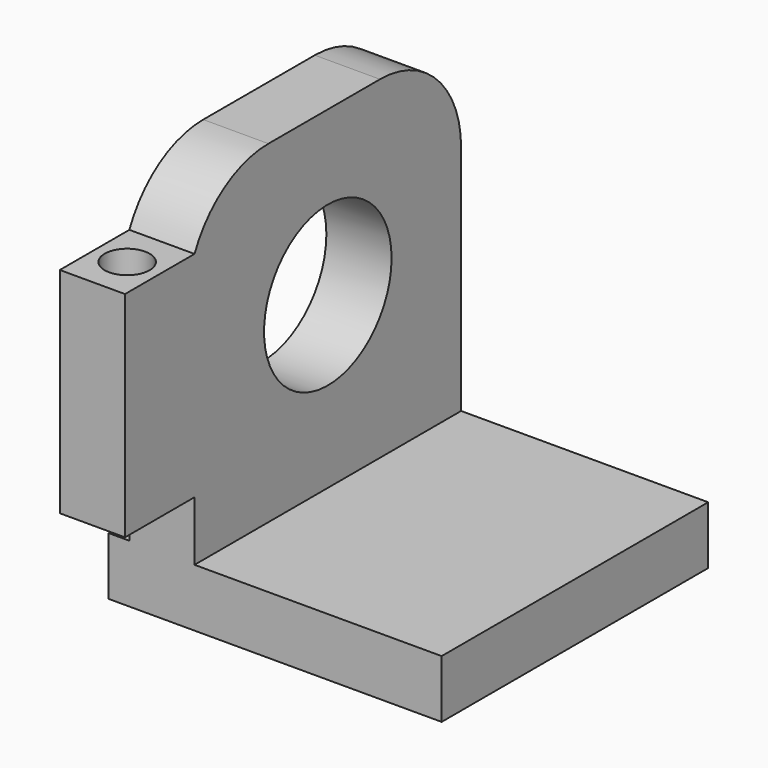
from build123d import *

# Parameters (mm, degrees)
F0_W         = 23
F0_H         = 23
F1_DEPTH     = 4
F2_W         = 4.5
F2_H         = 23
F3_DEPTH     = 23
F4_W         = 4.5
F4_H         = 14.783909363
F5_DEPTH     = 6
F7_D         = 11
F9_D         = 3.1
F10_T1_DEPTH = 39.5
F10_T3_DEPTH = 36.3734207923


# Not quite as in the source:
# - a fillet or chamfer that OpenCascade refuses, or shapes differently, is made with other operations: its cross-section is extruded or revolved along the edge and cut away or added


with BuildPart() as f1:
    # F0 (on Top) → F1 (new body)
    with BuildSketch(Plane.XY):
        Rectangle(F0_W, F0_H)
    extrude(amount=F1_DEPTH)

    # F2 (on face) → F3 (join)
    with BuildSketch(Plane.XY.offset(4)):
        with Locations((-7.8062060252, 0)):
            Rectangle(F2_W, F2_H)
    extrude(amount=F3_DEPTH)

    # F4 (on face) → F5 (join)
    with BuildSketch(Plane.XZ.offset(11.5)):
        with Locations((-7.8062060252, 15.5)):
            Rectangle(F4_W, F4_H)
    extrude(amount=F5_DEPTH)

    # F7 (through all)
    with Locations(Plane(origin=(-10.0562060252, 0, 0), x_dir=(0, -1, 0), z_dir=(-1, 0, 0))):
        with Locations((0, 15.7216731459)):
            Hole(F7_D / 2)

    # F9 (through all)
    with Locations(Plane.XY.offset(22.8919546815)):
        with Locations((-7.8062060252, -14.5)):
            Hole(F9_D / 2)

    # F10: fillet of radius 7 on 2 edges, made by hand

    # F10_s2 → F10_t1 (cut)
    with BuildSketch(Plane.YZ.offset(-27.5562060252)):
        with BuildLine():
            ThreePointArc((11.5, 20), (9.4497474683, 24.9497474683), (4.5, 27))
            Line((4.5, 27), (11.5, 27))
            Line((11.5, 27), (11.5, 20))
        make_face()
    extrude(amount=F10_T1_DEPTH, mode=Mode.SUBTRACT)

    # F10_s4 → F10_t3 (cut)
    with BuildSketch(Plane.YZ.offset(-25.9929164214)):
        with BuildLine():
            ThreePointArc((-5.1253158415, 27), (-8.9171700865, 25.8840327485), (-11.5, 22.8919546815))
            Line((-11.5, 22.8919546815), (-11.5, 27))
            Line((-11.5, 27), (-5.1253158415, 27))
        make_face()
    extrude(amount=F10_T3_DEPTH, mode=Mode.SUBTRACT)


solid = f1.part
